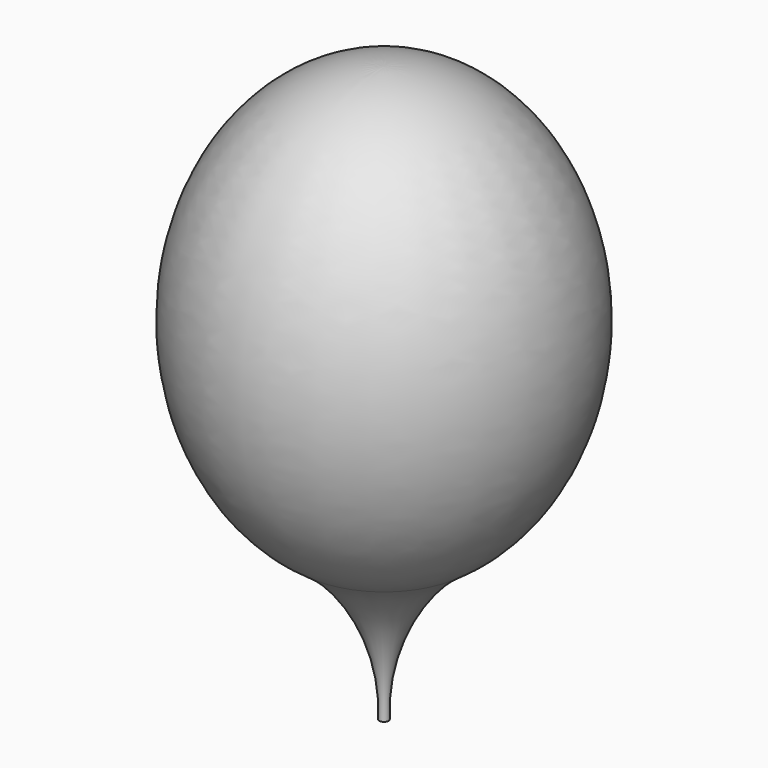
from build123d import *


with BuildPart() as f1:
    # F0 (on Right) → F1 (revolve)
    with BuildSketch(Plane.YZ):
        with BuildLine():
            Line((0, -500), (0, 500))
            add(Edge.make_bspline(
                [(0, 500), (-312.3467291674, 500), (-388.0678962691, 121.2133184546), (-463.7890633707, -257.5733630908), (-188.1559899699, -441.2293257169)],
                knots=[0, 0, 0, 1.3259300045, 1.3259300045, 2.651860009, 2.651860009, 2.651860009], degree=2, weights=[1, 0.7881708688, 1, 0.7881708688, 1]))
            ThreePointArc((-188.1559899699, -441.2293257169), (-53.3888950353, -592.8258288238), (-10.3115076199, -791.0378575325))
            Line((-10.3115076199, -791.0378575325), (0, -791.0378575325))
            Line((0, -791.0378575325), (0, -500))
        make_face()
    revolve(axis=Axis((0, 0, 0), (0, 0, 1)))


solid = f1.part
